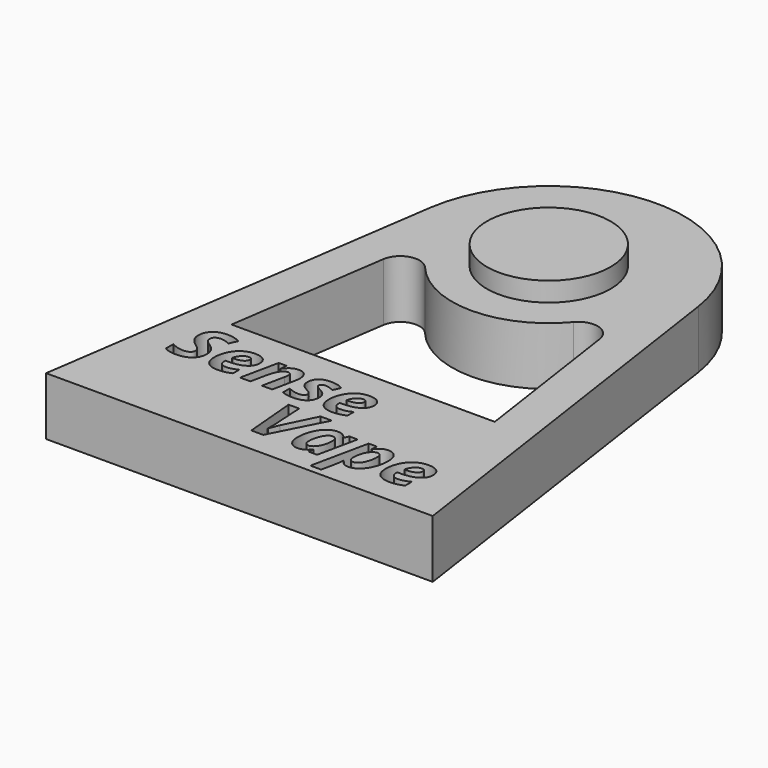
from build123d import *

# Parameters (mm, degrees)
F1_DEPTH       = 15
F2_R           = 16
F3_DEPTH       = 5
F4_R           = 16
F5_DEPTH       = 5
F7_DEPTH       = 15.001
F8_TEXT_SIZE   = 18.1077410593
F8_TEXT_SIZE_2 = 18.9374013677
F9_DEPTH       = 15.001


# Not quite as in the source:
# - Text() gives the source's letters only with a copy of the font that has no kerning and outlines rounded to 1/6400 em; it was checked with that copy


with BuildPart() as f1:
    # F0 (on Top) → F1 (new body)
    with BuildSketch(Plane.XY):
        with BuildLine():
            Line((-34.6314648142, 5.0657324071), (-50, -100))
            Line((-50, -100), (50, -100))
            Line((50, -100), (34.6314648142, 5.0657324071))
            ThreePointArc((34.6314648142, 5.0657324071), (0, 35), (-34.6314648142, 5.0657324071))
        make_face()
    extrude(amount=F1_DEPTH)

    # F2 (on face) → F3 (join)
    with BuildSketch(Plane.XY.offset(15)):
        Circle(F2_R)
    extrude(amount=F3_DEPTH)

    # F4 (on face) → F5 (cut)
    with BuildSketch(Plane(origin=(0, 0, 0), x_dir=(1, 0, 0), z_dir=(0, 0, -1))):
        Circle(F4_R)
    extrude(amount=-F5_DEPTH, mode=Mode.SUBTRACT)

    # F6 (on face) → F7 (cut, through all)
    with BuildSketch(Plane.XY.offset(15)):
        with BuildLine():
            Line((-27.9731383011, -18.5068509906), (-34.0425665143, -60))
            Line((-34.0425665143, -60), (34.0425665143, -60))
            Line((34.0425665143, -60), (27.9731383011, -18.5068509906))
            ThreePointArc((27.9731383011, -18.5068509906), (24.3849113929, -14.4187936118), (19.188155154, -16.0254392073))
            ThreePointArc((19.188155154, -16.0254392073), (0, -25), (-19.188155154, -16.0254392073))
            ThreePointArc((-19.188155154, -16.0254392073), (-24.3849113929, -14.4187936118), (-27.9731383011, -18.5068509906))
        make_face()
    extrude(amount=-F7_DEPTH, mode=Mode.SUBTRACT)

    # F8 (on face) → F9 (cut, through all)
    with BuildSketch(Plane.XY.offset(15)):
        with Locations((-38.2215323452, -77.0375735627)):
            Text('Sense', F8_TEXT_SIZE, font='Open Sans', font_style=FontStyle.BOLDITALIC, text_align=(TextAlign.LEFT, TextAlign.BOTTOM))
        with Locations((-4.8593882032, -93.6725025474)):
            Text('Vape', F8_TEXT_SIZE_2, font='Open Sans', font_style=FontStyle.BOLDITALIC, text_align=(TextAlign.LEFT, TextAlign.BOTTOM))
    extrude(amount=-F9_DEPTH, mode=Mode.SUBTRACT)


solid = f1.part
